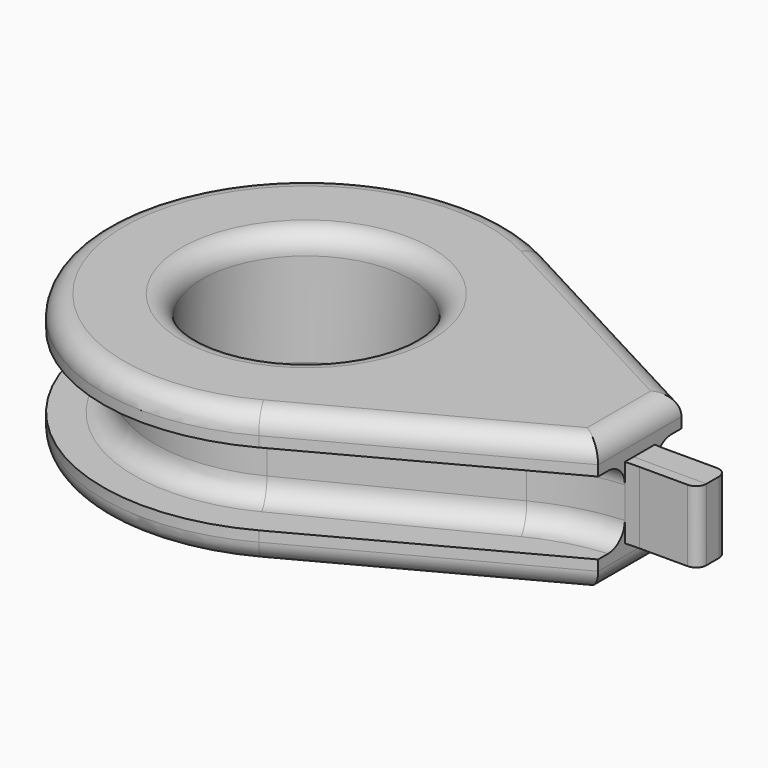
from build123d import *

# Parameters (mm, degrees)
F0_R          = 1
F1_DEPTH      = 1.3
F2_DEPTH      = 0.3
F3_START      = 1
F3_DEPTH      = 0.3
F4_W          = 0.15
F4_H          = 0.3062440047
F4_W_2        = 0.2115944407
F4_W_3        = 0.2297833452
F4_H_2        = 0.3057500289
F4_W_4        = 0.2163899079
F5_DEPTH      = 0.7
F6_T1_DEPTH   = 1.9872929377
F6_T3_DEPTH   = 1.9872929377
F6_T6_ANGLE   = 233.888716361
F6_T10_ANGLE  = 37.4026504782
F6_T15_ANGLE  = 37.4026504782
F6_T18_ANGLE  = 233.888716361
F6_T22_ANGLE  = 37.4026504782
F6_T27_ANGLE  = 37.4026504782
F6_T32_DEPTH  = 2
F6_T38_DEPTH  = 3.0860201082
F6_T41_ANGLE  = 236.2752472868
F6_T45_DEPTH  = 3.0860201082
F6_T52_DEPTH  = 3.0860201082
F6_T57_DEPTH  = 2
F6_T63_DEPTH  = 3.0860201082
F6_T66_ANGLE  = 236.2752472868
F6_T73_DEPTH  = 2
F6_T77_DEPTH  = 3.0860201082
F6_T84_DEPTH  = 2
F6_T88_DEPTH  = 3.0860201082
F6_T95_DEPTH  = 3.0860201082
F6_T99_DEPTH  = 2
F6_T106_DEPTH = 2
F6_T110_DEPTH = 3.0860201082


# Not quite as in the source:
# - a fillet or chamfer that OpenCascade refuses, or shapes differently, is made with other operations: its cross-section is extruded or revolved along the edge and cut away or added


with BuildPart() as f1:
    # F0 (on Top) → F1 (new body)
    with BuildSketch(Plane.XY):
        with BuildLine():
            ThreePointArc((2.4285975558, -0.3921060218), (2.8035605108, -0.2468573508), (3.2, -0.1795511441))
            ThreePointArc((3.2, -0.1795511441), (3.2673853882, -0.1761381098), (3.3348475558, -0.175))
            Line((3.3348475558, -0.175), (3.8, -0.175))
            ThreePointArc((3.8, -0.175), (3.8707106781, -0.1457106781), (3.9, -0.075))
            Line((3.9, -0.075), (3.9, 0))
            Line((3.9, 0), (3.9, 0.075))
            ThreePointArc((3.9, 0.075), (3.8707106781, 0.1457106781), (3.8, 0.175))
            Line((3.8, 0.175), (3.3348475558, 0.175))
            ThreePointArc((3.3348475558, 0.175), (3.2673853882, 0.1761381098), (3.2, 0.1795511441))
            ThreePointArc((3.2, 0.1795511441), (2.8035605108, 0.2468573508), (2.4285975558, 0.3921060218))
            Line((2.4285975558, 0.3921060218), (0.65703125, 1.2925981342))
            ThreePointArc((0.65703125, 1.2925981342), (-1.45, 0), (0.65703125, -1.2925981342))
            Line((0.65703125, -1.2925981342), (2.4285975558, -0.3921060218))
        make_face()
        Circle(F0_R, mode=Mode.SUBTRACT)
    extrude(amount=F1_DEPTH)

    # F0 (on Top) → F2 (join)
    with BuildSketch(Plane.XY):
        with BuildLine():
            ThreePointArc((2.4285975558, -0.3921060218), (2.8035605108, -0.2468573508), (3.2, -0.1795511441))
            ThreePointArc((3.2, -0.1795511441), (3.2673853882, -0.1761381098), (3.3348475558, -0.175))
            Line((3.3348475558, -0.175), (3.8, -0.175))
            ThreePointArc((3.8, -0.175), (3.8707106781, -0.1457106781), (3.9, -0.075))
            Line((3.9, -0.075), (3.9, 0))
            Line((3.9, 0), (3.9, 0.075))
            ThreePointArc((3.9, 0.075), (3.8707106781, 0.1457106781), (3.8, 0.175))
            Line((3.8, 0.175), (3.3348475558, 0.175))
            ThreePointArc((3.3348475558, 0.175), (3.2673853882, 0.1761381098), (3.2, 0.1795511441))
            ThreePointArc((3.2, 0.1795511441), (2.8035605108, 0.2468573508), (2.4285975558, 0.3921060218))
            Line((2.4285975558, 0.3921060218), (0.65703125, 1.2925981342))
            ThreePointArc((0.65703125, 1.2925981342), (-1.45, 0), (0.65703125, -1.2925981342))
            Line((0.65703125, -1.2925981342), (2.4285975558, -0.3921060218))
        make_face()
        Circle(F0_R, mode=Mode.SUBTRACT)
        with BuildLine():
            Line((3.2, -0.5), (3.2, -0.1795511441))
            ThreePointArc((3.2, -0.1795511441), (2.8035605108, -0.2468573508), (2.4285975558, -0.3921060218))
            Line((2.4285975558, -0.3921060218), (0.65703125, -1.2925981342))
            ThreePointArc((0.65703125, -1.2925981342), (-1.45, 0), (0.65703125, 1.2925981342))
            Line((0.65703125, 1.2925981342), (2.4285975558, 0.3921060218))
            ThreePointArc((2.4285975558, 0.3921060218), (2.8035605108, 0.2468573508), (3.2, 0.1795511441))
            Line((3.2, 0.1795511441), (3.2, 0.5))
            Line((3.2, 0.5), (0.9196025162, 1.7195438966))
            ThreePointArc((0.9196025162, 1.7195438966), (-1.95, 0), (0.9196025162, -1.7195438966))
            Line((0.9196025162, -1.7195438966), (3.2, -0.5))
        make_face()
    extrude(amount=F2_DEPTH)

    # F0 (on Top) → F3 (join)
    with BuildSketch(Plane.XY.offset(F3_START)):
        with BuildLine():
            ThreePointArc((2.4285975558, -0.3921060218), (2.8035605108, -0.2468573508), (3.2, -0.1795511441))
            ThreePointArc((3.2, -0.1795511441), (3.2673853882, -0.1761381098), (3.3348475558, -0.175))
            Line((3.3348475558, -0.175), (3.8, -0.175))
            ThreePointArc((3.8, -0.175), (3.8707106781, -0.1457106781), (3.9, -0.075))
            Line((3.9, -0.075), (3.9, 0))
            Line((3.9, 0), (3.9, 0.075))
            ThreePointArc((3.9, 0.075), (3.8707106781, 0.1457106781), (3.8, 0.175))
            Line((3.8, 0.175), (3.3348475558, 0.175))
            ThreePointArc((3.3348475558, 0.175), (3.2673853882, 0.1761381098), (3.2, 0.1795511441))
            ThreePointArc((3.2, 0.1795511441), (2.8035605108, 0.2468573508), (2.4285975558, 0.3921060218))
            Line((2.4285975558, 0.3921060218), (0.65703125, 1.2925981342))
            ThreePointArc((0.65703125, 1.2925981342), (-1.45, 0), (0.65703125, -1.2925981342))
            Line((0.65703125, -1.2925981342), (2.4285975558, -0.3921060218))
        make_face()
        Circle(F0_R, mode=Mode.SUBTRACT)
        with BuildLine():
            Line((3.2, -0.5), (3.2, -0.1795511441))
            ThreePointArc((3.2, -0.1795511441), (2.8035605108, -0.2468573508), (2.4285975558, -0.3921060218))
            Line((2.4285975558, -0.3921060218), (0.65703125, -1.2925981342))
            ThreePointArc((0.65703125, -1.2925981342), (-1.45, 0), (0.65703125, 1.2925981342))
            Line((0.65703125, 1.2925981342), (2.4285975558, 0.3921060218))
            ThreePointArc((2.4285975558, 0.3921060218), (2.8035605108, 0.2468573508), (3.2, 0.1795511441))
            Line((3.2, 0.1795511441), (3.2, 0.5))
            Line((3.2, 0.5), (0.9196025162, 1.7195438966))
            ThreePointArc((0.9196025162, 1.7195438966), (-1.95, 0), (0.9196025162, -1.7195438966))
            Line((0.9196025162, -1.7195438966), (3.2, -0.5))
        make_face()
    extrude(amount=F3_DEPTH)

    # F4 (on face) → F5 (cut)
    with BuildSketch(Plane.YZ.offset(3.9)):
        Polygon((-0.075, 1.3), (-0.2913899079, 1.3), (-0.3079036542, 0.9937559953), (-0.075, 0.9937559953), align=None)
        with Locations((0, 1.1468779976)):
            Rectangle(F4_W, F4_H)
        with Locations((0.1807972203, 1.1468779976)):
            Rectangle(F4_W_2, F4_H)
        with Locations((0.1898916726, 0.1528750145)):
            Rectangle(F4_W_3, F4_H_2)
        with Locations((0, 0.1528750145)):
            Rectangle(F4_W, F4_H_2)
        with Locations((-0.183194954, 0.1528750145)):
            Rectangle(F4_W_4, F4_H_2)
    extrude(amount=-F5_DEPTH, mode=Mode.SUBTRACT)

    # F6: fillet of radius 0.2 on 14 edges, made by hand

    # F6_s2 → F6_t1 (join)
    with BuildSketch(Plane(origin=(0, 0, 0), x_dir=(0, 0, 1), z_dir=(0.8914469891, 0.453125, 0))):
        with BuildLine():
            ThreePointArc((0.3, 1.65), (0.3585786438, 1.5085786438), (0.5, 1.45))
            Line((0.5, 1.45), (0.5, 1.446))
            Line((0.5, 1.446), (0.296, 1.446))
            Line((0.296, 1.446), (0.296, 1.65))
            Line((0.296, 1.65), (0.3, 1.65))
        make_face()
        with BuildLine():
            ThreePointArc((1, 1.65), (0.9414213562, 1.5085786438), (0.8, 1.45))
            Line((0.8, 1.45), (0.8, 1.446))
            Line((0.8, 1.446), (1.004, 1.446))
            Line((1.004, 1.446), (1.004, 1.65))
            Line((1.004, 1.65), (1, 1.65))
        make_face()
    extrude(amount=F6_T1_DEPTH)

    # F6_s4 → F6_t3 (join)
    with BuildSketch(Plane(origin=(1.7715663058, -0.9004921124, 0), x_dir=(0, 0, 1), z_dir=(-0.8914469891, 0.453125, 0))):
        with BuildLine():
            ThreePointArc((1, 1.65), (0.9414213562, 1.5085786438), (0.8, 1.45))
            Line((0.8, 1.45), (0.8, 1.446))
            Line((0.8, 1.446), (1.004, 1.446))
            Line((1.004, 1.446), (1.004, 1.65))
            Line((1.004, 1.65), (1, 1.65))
        make_face()
        with BuildLine():
            ThreePointArc((0.3, 1.65), (0.3585786438, 1.5085786438), (0.5, 1.45))
            Line((0.5, 1.45), (0.5, 1.446))
            Line((0.5, 1.446), (0.296, 1.446))
            Line((0.296, 1.446), (0.296, 1.65))
            Line((0.296, 1.65), (0.3, 1.65))
        make_face()
    extrude(amount=F6_T3_DEPTH)

    # F6_s5 → F6_t6 (revolve)
    with BuildSketch(Plane(origin=(0, 0, 0), x_dir=(0, 0, 1), z_dir=(0.8914469891, 0.453125, 0))):
        with BuildLine():
            ThreePointArc((1, 1.65), (0.9414213562, 1.5085786438), (0.8, 1.45))
            Line((0.8, 1.45), (0.8, 1.446))
            Line((0.8, 1.446), (1.004, 1.446))
            Line((1.004, 1.446), (1.004, 1.65))
            Line((1.004, 1.65), (1, 1.65))
        make_face()
    revolve(axis=Axis((0, 0, 1), (0, 0, -1)), revolution_arc=F6_T6_ANGLE)


with BuildPart() as f6_tool8:
    # F6_s9 → F6_t10 (revolve)
    with BuildSketch(Plane(origin=(1.7715663058, 0.9004921124, 0), x_dir=(0, 0, 1), z_dir=(-0.8914469891, -0.453125, 0))):
        with BuildLine():
            ThreePointArc((1, -1.65), (0.9414213562, -1.5085786438), (0.8, -1.45))
            Line((0.8, -1.45), (0.8, -1.446))
            Line((0.8, -1.446), (1.004, -1.446))
            Line((1.004, -1.446), (1.004, -1.65))
            Line((1.004, -1.65), (1, -1.65))
        make_face()
    revolve(axis=Axis((3.3348475558, -2.175, 1), (0, 0, -1)), revolution_arc=F6_T10_ANGLE)

    split(bisect_by=Plane.YZ.offset(3.2), keep=Keep.BOTTOM)


with BuildPart() as f1_1:
    add(f1.part)

    # F6_t7: union F6_tool8
    add(f6_tool8.part)


with BuildPart() as f6_tool13:
    # F6_s14 → F6_t15 (revolve)
    with BuildSketch(Plane(origin=(3.6132129184, 0.666949259, 0), x_dir=(0, 0, 1), z_dir=(0.983387303, 0.1815197299, 0))):
        with BuildLine():
            ThreePointArc((1, 0.2664732437), (0.9414213562, 0.4078945999), (0.8, 0.4664732437))
            Line((0.8, 0.4664732437), (0.8, 0.4704732437))
            Line((0.8, 0.4704732437), (1.004, 0.4704732437))
            Line((1.004, 0.4704732437), (1.004, 0.2664732437))
            Line((1.004, 0.2664732437), (1, 0.2664732437))
        make_face()
    revolve(axis=Axis((3.3348475558, 2.175, 1), (0, 0, -1)), revolution_arc=F6_T15_ANGLE)

    split(bisect_by=Plane.YZ.offset(3.2), keep=Keep.BOTTOM)


with BuildPart() as f1_2:
    add(f1_1.part)

    # F6_t12: union F6_tool13
    add(f6_tool13.part)

    # F6_s17 → F6_t18 (revolve)
    with BuildSketch(Plane(origin=(0, 0, 0), x_dir=(0, 0, 1), z_dir=(0.8914469891, 0.453125, 0))):
        with BuildLine():
            ThreePointArc((0.3, 1.65), (0.3585786438, 1.5085786438), (0.5, 1.45))
            Line((0.5, 1.45), (0.5, 1.446))
            Line((0.5, 1.446), (0.296, 1.446))
            Line((0.296, 1.446), (0.296, 1.65))
            Line((0.296, 1.65), (0.3, 1.65))
        make_face()
    revolve(axis=Axis((0, 0, 0.3), (0, 0, -1)), revolution_arc=F6_T18_ANGLE)


with BuildPart() as f6_tool20:
    # F6_s21 → F6_t22 (revolve)
    with BuildSketch(Plane(origin=(1.7715663058, 0.9004921124, 0), x_dir=(0, 0, 1), z_dir=(-0.8914469891, -0.453125, 0))):
        with BuildLine():
            ThreePointArc((0.3, -1.65), (0.3585786438, -1.5085786438), (0.5, -1.45))
            Line((0.5, -1.45), (0.5, -1.446))
            Line((0.5, -1.446), (0.296, -1.446))
            Line((0.296, -1.446), (0.296, -1.65))
            Line((0.296, -1.65), (0.3, -1.65))
        make_face()
    revolve(axis=Axis((3.3348475558, -2.175, 0.3), (0, 0, -1)), revolution_arc=F6_T22_ANGLE)

    split(bisect_by=Plane.YZ.offset(3.2), keep=Keep.BOTTOM)


with BuildPart() as f1_3:
    add(f1_2.part)

    # F6_t19: union F6_tool20
    add(f6_tool20.part)


with BuildPart() as f6_tool25:
    # F6_s26 → F6_t27 (revolve)
    with BuildSketch(Plane(origin=(3.6132129184, 0.666949259, 0), x_dir=(0, 0, 1), z_dir=(0.983387303, 0.1815197299, 0))):
        with BuildLine():
            ThreePointArc((0.5, 0.4664732437), (0.3585786438, 0.4078945999), (0.3, 0.2664732437))
            Line((0.3, 0.2664732437), (0.296, 0.2664732437))
            Line((0.296, 0.2664732437), (0.296, 0.4704732437))
            Line((0.296, 0.4704732437), (0.5, 0.4704732437))
            Line((0.5, 0.4704732437), (0.5, 0.4664732437))
        make_face()
    revolve(axis=Axis((3.3348475558, 2.175, 0.3), (0, 0, -1)), revolution_arc=F6_T27_ANGLE)

    split(bisect_by=Plane.YZ.offset(3.2), keep=Keep.BOTTOM)


with BuildPart() as f1_4:
    add(f1_3.part)

    # F6_t24: union F6_tool25
    add(f6_tool25.part)


with BuildPart() as f6_tool30:
    # F6_s31 → F6_t32 (new body)
    with BuildSketch(Plane.XZ.offset(1)):
        with BuildLine():
            ThreePointArc((3, 1.3), (3.1414213562, 1.2414213562), (3.2, 1.1))
            Line((3.2, 1.1), (3.204, 1.1))
            Line((3.204, 1.1), (3.204, 1.304))
            Line((3.204, 1.304), (3, 1.304))
            Line((3, 1.304), (3, 1.3))
        make_face()
    extrude(amount=-F6_T32_DEPTH)

    split(bisect_by=Plane(origin=(0.9196025162, -1.7195438966, 0), x_dir=(0, 0, 1), z_dir=(-0.4715910339, 0.8818173829, 0)), keep=Keep.TOP)

    split(bisect_by=Plane(origin=(0.9196025162, 1.7195438966, 0), x_dir=(0, 0, 1), z_dir=(-0.4715910339, -0.8818173829, 0)), keep=Keep.TOP)


with BuildPart() as f1_5:
    add(f1_4.part)

    # F6_t29: cut F6_tool30
    add(f6_tool30.part, mode=Mode.SUBTRACT)


with BuildPart() as f6_tool36:
    # F6_s37 → F6_t38 (new body)
    with BuildSketch(Plane(origin=(2.7213061753, -1.4553394135, 0), x_dir=(0, 0, 1), z_dir=(-0.8818173829, 0.4715910339, 0))):
        with BuildLine():
            ThreePointArc((1.3, 1.75), (1.2414213562, 1.8914213562), (1.1, 1.95))
            Line((1.1, 1.95), (1.1, 1.954))
            Line((1.1, 1.954), (1.304, 1.954))
            Line((1.304, 1.954), (1.304, 1.75))
            Line((1.304, 1.75), (1.3, 1.75))
        make_face()
    extrude(amount=F6_T38_DEPTH)

    split(bisect_by=Plane.YZ.offset(3.2), keep=Keep.BOTTOM)


with BuildPart() as f1_6:
    add(f1_5.part)

    # F6_t35: cut F6_tool36
    add(f6_tool36.part, mode=Mode.SUBTRACT)

    # F6_s40 → F6_t41 (revolve, cut)
    with BuildSketch(Plane(origin=(0, 0, 0), x_dir=(0, 0, 1), z_dir=(0.8818173829, -0.4715910339, 0))):
        with BuildLine():
            ThreePointArc((1.3, -1.75), (1.2414213562, -1.8914213562), (1.1, -1.95))
            Line((1.1, -1.95), (1.1, -1.954))
            Line((1.1, -1.954), (1.304, -1.954))
            Line((1.304, -1.954), (1.304, -1.75))
            Line((1.304, -1.75), (1.3, -1.75))
        make_face()
    revolve(axis=Axis((0, 0, 1.3), (0, 0, 1)), revolution_arc=F6_T41_ANGLE, mode=Mode.SUBTRACT)


with BuildPart() as f6_tool43:
    # F6_s44 → F6_t45 (new body)
    with BuildSketch(Plane(origin=(0, 0, 0), x_dir=(0, 0, 1), z_dir=(0.8818173829, 0.4715910339, 0))):
        with BuildLine():
            ThreePointArc((1.3, 1.75), (1.2414213562, 1.8914213562), (1.1, 1.95))
            Line((1.1, 1.95), (1.1, 1.954))
            Line((1.1, 1.954), (1.304, 1.954))
            Line((1.304, 1.954), (1.304, 1.75))
            Line((1.304, 1.75), (1.3, 1.75))
        make_face()
    extrude(amount=F6_T45_DEPTH)

    split(bisect_by=Plane.YZ.offset(3.2), keep=Keep.BOTTOM)


with BuildPart() as f1_7:
    add(f1_6.part)

    # F6_t42: cut F6_tool43
    add(f6_tool43.part, mode=Mode.SUBTRACT)

    # F6_s47 → F6_t48 (revolve, cut)
    with BuildSketch(Plane.XZ):
        with BuildLine():
            ThreePointArc((1, 1.1), (1.0585786438, 1.2414213562), (1.2, 1.3))
            Line((1.2, 1.3), (1.2, 1.304))
            Line((1.2, 1.304), (0.996, 1.304))
            Line((0.996, 1.304), (0.996, 1.1))
            Line((0.996, 1.1), (1, 1.1))
        make_face()
    revolve(axis=Axis((0, 0, 1.3), (0, 0, 1)), mode=Mode.SUBTRACT)


with BuildPart() as f6_tool50:
    # F6_s51 → F6_t52 (new body)
    with BuildSketch(Plane(origin=(0, 0, 0), x_dir=(0, 0, 1), z_dir=(0.8818173829, 0.4715910339, 0))):
        with BuildLine():
            ThreePointArc((0, 1.75), (0.0585786438, 1.8914213562), (0.2, 1.95))
            Line((0.2, 1.95), (0.2, 1.954))
            Line((0.2, 1.954), (-0.004, 1.954))
            Line((-0.004, 1.954), (-0.004, 1.75))
            Line((-0.004, 1.75), (0, 1.75))
        make_face()
    extrude(amount=F6_T52_DEPTH)

    split(bisect_by=Plane.YZ.offset(3.2), keep=Keep.BOTTOM)


with BuildPart() as f1_8:
    add(f1_7.part)

    # F6_t49: cut F6_tool50
    add(f6_tool50.part, mode=Mode.SUBTRACT)


with BuildPart() as f6_tool55:
    # F6_s56 → F6_t57 (new body)
    with BuildSketch(Plane.XZ.offset(-1)):
        with BuildLine():
            ThreePointArc((3, 0), (3.1414213562, 0.0585786438), (3.2, 0.2))
            Line((3.2, 0.2), (3.204, 0.2))
            Line((3.204, 0.2), (3.204, -0.004))
            Line((3.204, -0.004), (3, -0.004))
            Line((3, -0.004), (3, 0))
        make_face()
    extrude(amount=F6_T57_DEPTH)

    split(bisect_by=Plane(origin=(0.9196025162, 1.7195438966, 0), x_dir=(0, 0, 1), z_dir=(-0.4715910339, -0.8818173829, 0)), keep=Keep.TOP)

    split(bisect_by=Plane(origin=(0.9196025162, -1.7195438966, 0), x_dir=(0, 0, 1), z_dir=(-0.4715910339, 0.8818173829, 0)), keep=Keep.TOP)


with BuildPart() as f1_9:
    add(f1_8.part)

    # F6_t54: cut F6_tool55
    add(f6_tool55.part, mode=Mode.SUBTRACT)


with BuildPart() as f6_tool61:
    # F6_s62 → F6_t63 (new body)
    with BuildSketch(Plane(origin=(2.7213061753, -1.4553394135, 0), x_dir=(0, 0, 1), z_dir=(-0.8818173829, 0.4715910339, 0))):
        with BuildLine():
            ThreePointArc((0, 1.75), (0.0585786438, 1.8914213562), (0.2, 1.95))
            Line((0.2, 1.95), (0.2, 1.954))
            Line((0.2, 1.954), (-0.004, 1.954))
            Line((-0.004, 1.954), (-0.004, 1.75))
            Line((-0.004, 1.75), (0, 1.75))
        make_face()
    extrude(amount=F6_T63_DEPTH)

    split(bisect_by=Plane.YZ.offset(3.2), keep=Keep.BOTTOM)


with BuildPart() as f1_10:
    add(f1_9.part)

    # F6_t60: cut F6_tool61
    add(f6_tool61.part, mode=Mode.SUBTRACT)

    # F6_s65 → F6_t66 (revolve, cut)
    with BuildSketch(Plane(origin=(0, 0, 0), x_dir=(0, 0, 1), z_dir=(0.8818173829, -0.4715910339, 0))):
        with BuildLine():
            ThreePointArc((0, -1.75), (0.0585786438, -1.8914213562), (0.2, -1.95))
            Line((0.2, -1.95), (0.2, -1.954))
            Line((0.2, -1.954), (-0.004, -1.954))
            Line((-0.004, -1.954), (-0.004, -1.75))
            Line((-0.004, -1.75), (0, -1.75))
        make_face()
    revolve(axis=Axis((0, 0, 0), (0, 0, 1)), revolution_arc=F6_T66_ANGLE, mode=Mode.SUBTRACT)

    # F6_s67 → F6_t68 (revolve, cut)
    with BuildSketch(Plane.XZ):
        with BuildLine():
            ThreePointArc((1.2, 0), (1.0585786438, 0.0585786438), (1, 0.2))
            Line((1, 0.2), (0.996, 0.2))
            Line((0.996, 0.2), (0.996, -0.004))
            Line((0.996, -0.004), (1.2, -0.004))
            Line((1.2, -0.004), (1.2, 0))
        make_face()
    revolve(axis=Axis((0, 0, 0), (0, 0, 1)), mode=Mode.SUBTRACT)


with BuildPart() as f6_tool71:
    # F6_s72 → F6_t73 (new body)
    with BuildSketch(Plane.XZ.offset(1)):
        with BuildLine():
            ThreePointArc((3, 1.3), (3.1414213562, 1.2414213562), (3.2, 1.1))
            Line((3.2, 1.1), (3.204, 1.1))
            Line((3.204, 1.1), (3.204, 1.304))
            Line((3.204, 1.304), (3, 1.304))
            Line((3, 1.304), (3, 1.3))
        make_face()
    extrude(amount=-F6_T73_DEPTH)

    split(bisect_by=Plane(origin=(0.9196025162, -1.7195438966, 0), x_dir=(0, 0, 1), z_dir=(0.4715910339, -0.8818173829, 0)), keep=Keep.TOP)


with BuildPart() as f6_tool75:
    # F6_s76 → F6_t77 (new body)
    with BuildSketch(Plane(origin=(0, 0, 0), x_dir=(0, 0, 1), z_dir=(0.8818173829, 0.4715910339, 0))):
        with BuildLine():
            ThreePointArc((1.3, 1.75), (1.2414213562, 1.8914213562), (1.1, 1.95))
            Line((1.1, 1.95), (1.1, 1.954))
            Line((1.1, 1.954), (1.304, 1.954))
            Line((1.304, 1.954), (1.304, 1.75))
            Line((1.304, 1.75), (1.3, 1.75))
        make_face()
    extrude(amount=F6_T77_DEPTH)

    split(bisect_by=Plane.YZ.offset(3.2), keep=Keep.TOP)


with BuildPart() as f6_tool71_1:
    add(f6_tool71.part)

    # F6_t79: intersect F6_tool75
    add(f6_tool75.part, mode=Mode.INTERSECT)


with BuildPart() as f1_11:
    add(f1_10.part)

    # F6_t69: cut F6_tool71
    add(f6_tool71_1.part, mode=Mode.SUBTRACT)


with BuildPart() as f6_tool82:
    # F6_s83 → F6_t84 (new body)
    with BuildSketch(Plane.XZ.offset(1)):
        with BuildLine():
            ThreePointArc((3, 1.3), (3.1414213562, 1.2414213562), (3.2, 1.1))
            Line((3.2, 1.1), (3.204, 1.1))
            Line((3.204, 1.1), (3.204, 1.304))
            Line((3.204, 1.304), (3, 1.304))
            Line((3, 1.304), (3, 1.3))
        make_face()
    extrude(amount=-F6_T84_DEPTH)

    split(bisect_by=Plane(origin=(0.9196025162, 1.7195438966, 0), x_dir=(0, 0, 1), z_dir=(0.4715910339, 0.8818173829, 0)), keep=Keep.TOP)


with BuildPart() as f6_tool86:
    # F6_s87 → F6_t88 (new body)
    with BuildSketch(Plane(origin=(2.7213061753, -1.4553394135, 0), x_dir=(0, 0, 1), z_dir=(-0.8818173829, 0.4715910339, 0))):
        with BuildLine():
            ThreePointArc((1.3, 1.75), (1.2414213562, 1.8914213562), (1.1, 1.95))
            Line((1.1, 1.95), (1.1, 1.954))
            Line((1.1, 1.954), (1.304, 1.954))
            Line((1.304, 1.954), (1.304, 1.75))
            Line((1.304, 1.75), (1.3, 1.75))
        make_face()
    extrude(amount=F6_T88_DEPTH)

    split(bisect_by=Plane.YZ.offset(3.2), keep=Keep.TOP)


with BuildPart() as f6_tool82_1:
    add(f6_tool82.part)

    # F6_t90: intersect F6_tool86
    add(f6_tool86.part, mode=Mode.INTERSECT)


with BuildPart() as f1_12:
    add(f1_11.part)

    # F6_t80: cut F6_tool82
    add(f6_tool82_1.part, mode=Mode.SUBTRACT)


with BuildPart() as f6_tool93:
    # F6_s94 → F6_t95 (new body)
    with BuildSketch(Plane(origin=(0, 0, 0), x_dir=(0, 0, 1), z_dir=(0.8818173829, 0.4715910339, 0))):
        with BuildLine():
            ThreePointArc((0, 1.75), (0.0585786438, 1.8914213562), (0.2, 1.95))
            Line((0.2, 1.95), (0.2, 1.954))
            Line((0.2, 1.954), (-0.004, 1.954))
            Line((-0.004, 1.954), (-0.004, 1.75))
            Line((-0.004, 1.75), (0, 1.75))
        make_face()
    extrude(amount=F6_T95_DEPTH)

    split(bisect_by=Plane.YZ.offset(3.2), keep=Keep.TOP)


with BuildPart() as f6_tool97:
    # F6_s98 → F6_t99 (new body)
    with BuildSketch(Plane.XZ.offset(-1)):
        with BuildLine():
            ThreePointArc((3, 0), (3.1414213562, 0.0585786438), (3.2, 0.2))
            Line((3.2, 0.2), (3.204, 0.2))
            Line((3.204, 0.2), (3.204, -0.004))
            Line((3.204, -0.004), (3, -0.004))
            Line((3, -0.004), (3, 0))
        make_face()
    extrude(amount=F6_T99_DEPTH)

    split(bisect_by=Plane(origin=(0.9196025162, -1.7195438966, 0), x_dir=(0, 0, 1), z_dir=(0.4715910339, -0.8818173829, 0)), keep=Keep.TOP)


with BuildPart() as f6_tool93_1:
    add(f6_tool93.part)

    # F6_t101: intersect F6_tool97
    add(f6_tool97.part, mode=Mode.INTERSECT)


with BuildPart() as f1_13:
    add(f1_12.part)

    # F6_t91: cut F6_tool93
    add(f6_tool93_1.part, mode=Mode.SUBTRACT)


with BuildPart() as f6_tool104:
    # F6_s105 → F6_t106 (new body)
    with BuildSketch(Plane.XZ.offset(-1)):
        with BuildLine():
            ThreePointArc((3, 0), (3.1414213562, 0.0585786438), (3.2, 0.2))
            Line((3.2, 0.2), (3.204, 0.2))
            Line((3.204, 0.2), (3.204, -0.004))
            Line((3.204, -0.004), (3, -0.004))
            Line((3, -0.004), (3, 0))
        make_face()
    extrude(amount=F6_T106_DEPTH)

    split(bisect_by=Plane(origin=(0.9196025162, 1.7195438966, 0), x_dir=(0, 0, 1), z_dir=(0.4715910339, 0.8818173829, 0)), keep=Keep.TOP)


with BuildPart() as f6_tool108:
    # F6_s109 → F6_t110 (new body)
    with BuildSketch(Plane(origin=(2.7213061753, -1.4553394135, 0), x_dir=(0, 0, 1), z_dir=(-0.8818173829, 0.4715910339, 0))):
        with BuildLine():
            ThreePointArc((0, 1.75), (0.0585786438, 1.8914213562), (0.2, 1.95))
            Line((0.2, 1.95), (0.2, 1.954))
            Line((0.2, 1.954), (-0.004, 1.954))
            Line((-0.004, 1.954), (-0.004, 1.75))
            Line((-0.004, 1.75), (0, 1.75))
        make_face()
    extrude(amount=F6_T110_DEPTH)

    split(bisect_by=Plane.YZ.offset(3.2), keep=Keep.TOP)


with BuildPart() as f6_tool104_1:
    add(f6_tool104.part)

    # F6_t112: intersect F6_tool108
    add(f6_tool108.part, mode=Mode.INTERSECT)


with BuildPart() as f1_14:
    add(f1_13.part)

    # F6_t102: cut F6_tool104
    add(f6_tool104_1.part, mode=Mode.SUBTRACT)


solid = f1_14.part
